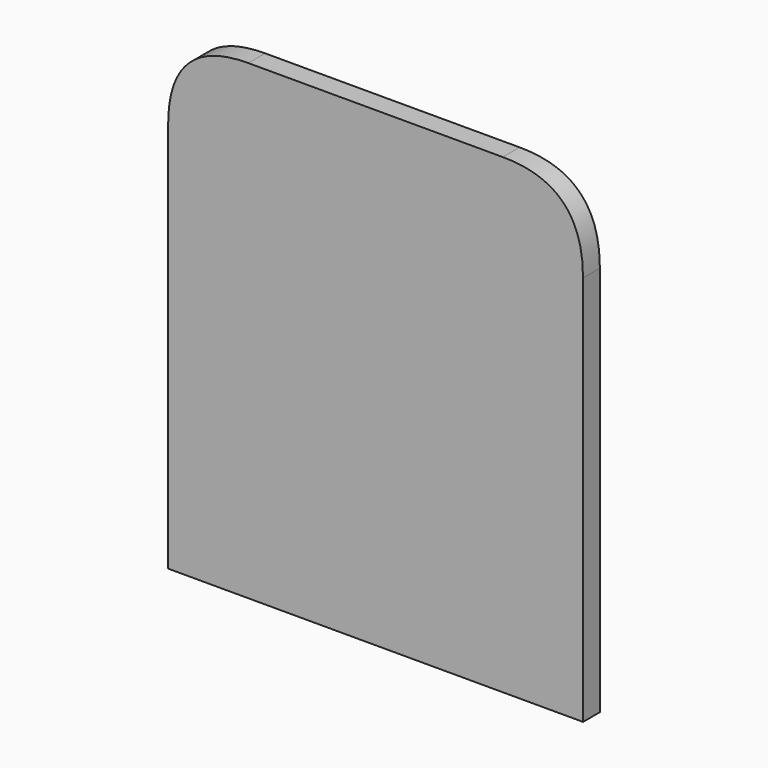
from build123d import *

# Parameters (mm, degrees)
F0_W        = 394
F0_H        = 447.4
F1_DEPTH    = 20
F2_T1_DEPTH = 401


# Not quite as in the source:
# - a fillet or chamfer that OpenCascade refuses, or shapes differently, is made with other operations: its cross-section is extruded or revolved along the edge and cut away or added


with BuildPart() as f1:
    # F0 (on Front) → F1 (new body)
    with BuildSketch(Plane.XZ):
        with Locations((33.1907154322, 42.8427122533)):
            Rectangle(F0_W, F0_H)
    extrude(amount=F1_DEPTH)

    # F2: fillet of radius 76.2 on 2 edges, made by hand

    # F2_s2 → F2_t1 (cut)
    with BuildSketch(Plane.XZ.offset(-190.5)):
        with BuildLine():
            add(Edge.make_bspline(
                [(153.9907154322, 266.5427122533), (230.1907154322, 266.5427122533), (230.1907154322, 190.3427122533)],
                knots=[0, 0, 0, 1, 1, 1], degree=2, weights=[1, 1, 1]))
            Line((230.1907154322, 190.3427122533), (230.1907154322, 266.5427122533))
            Line((230.1907154322, 266.5427122533), (153.9907154322, 266.5427122533))
        make_face()
        with BuildLine():
            add(Edge.make_bspline(
                [(-87.6092845678, 266.5427122533), (-163.8092845678, 266.5427122533), (-163.8092845678, 190.3427122533)],
                knots=[0, 0, 0, 1, 1, 1], degree=2, weights=[1, 1, 1]))
            Line((-163.8092845678, 190.3427122533), (-163.8092845678, 266.5427122533))
            Line((-163.8092845678, 266.5427122533), (-87.6092845678, 266.5427122533))
        make_face()
    extrude(amount=F2_T1_DEPTH, mode=Mode.SUBTRACT)


solid = f1.part
